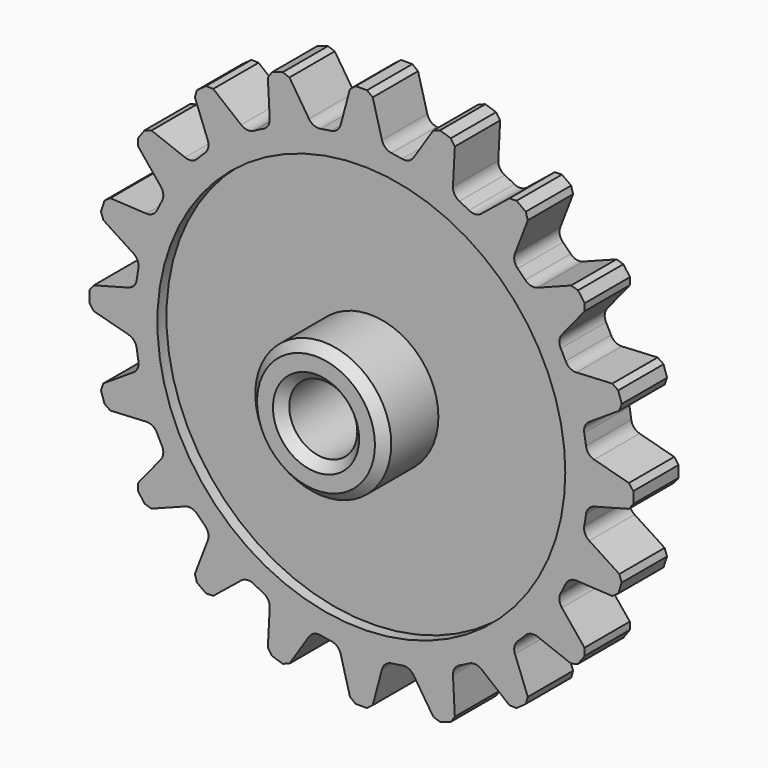
from build123d import *

# Parameters (mm, degrees)
F0_R            = 100
F1_DEPTH        = 25
F3_DEPTH        = 25
F3_COPIES_COUNT = 20
F4_R            = 5
F5_SIZE         = 2
F6_R            = 90
F7_DEPTH        = 5
F8_R            = 30
F9_DEPTH        = 30
F10_R           = 15
F11_DEPTH       = 50.001
F12_SIZE        = 4


# Not quite as in the source:
# - a pattern or mirror of a feature is missing from the dataset's text; its kind, count and spacing are read off the source's solid


with BuildPart() as f1:
    # F0 (on Front) → F1 (new body)
    with BuildSketch(Plane.XZ):
        Circle(F0_R)
    extrude(amount=F1_DEPTH)

    # F2 (on face) → F3 (join, through all)
    with BuildSketch(Plane.XZ.offset(25)):
        with BuildLine():
            Line((-4.5, 120), (-9.9931095726, 99.4994359837))
            ThreePointArc((-9.9931095726, 99.4994359837), (0, 100), (9.9931095726, 99.4994359837))
            Line((9.9931095726, 99.4994359837), (4.5, 120))
            Line((4.5, 120), (-4.5, 120))
        make_face()
    f3 = extrude(amount=-F3_DEPTH)

    # F3_copies: F3 ×20 about axis
    f3_copies_axis = Axis((0, 0, 0), (0, 1, 0))
    for i in range(1, F3_COPIES_COUNT):
        add(f3.rotate(f3_copies_axis, i * 360 / F3_COPIES_COUNT))

    # F4
    f4_edges = [f1.edges().sort_by_distance(p)[0] for p in [
        (9.99311, -12.5, 99.499436),
        (-9.99311, -12.5, 99.499436),
        (-21.243005, -12.5, 97.717628),
        (-50.399706, -12.5, 86.370537),
        (-40.251029, -12.5, 91.541546),
        (-66.568897, -12.5, 74.622932),
        (-74.622932, -12.5, 66.568897),
        (-86.370537, -12.5, 50.399706),
        (-91.541546, -12.5, 40.251029),
        (-97.717628, -12.5, 21.243005),
        (-99.499436, -12.5, 9.99311),
        (-99.499436, -12.5, -9.99311),
        (-97.717628, -12.5, -21.243005),
        (-91.541546, -12.5, -40.251029),
        (-86.370537, -12.5, -50.399706),
        (-74.622932, -12.5, -66.568897),
        (-66.568897, -12.5, -74.622932),
        (-50.399706, -12.5, -86.370537),
        (-40.251029, -12.5, -91.541546),
        (-21.243005, -12.5, -97.717628),
        (-9.99311, -12.5, -99.499436),
        (9.99311, -12.5, -99.499436),
        (21.243005, -12.5, -97.717628),
        (40.251029, -12.5, -91.541546),
        (50.399706, -12.5, -86.370537),
        (66.568897, -12.5, -74.622932),
        (74.622932, -12.5, -66.568897),
        (86.370537, -12.5, -50.399706),
        (91.541546, -12.5, -40.251029),
        (97.717628, -12.5, -21.243005),
        (99.499436, -12.5, -9.99311),
        (99.499436, -12.5, 9.99311),
        (97.717628, -12.5, 21.243005),
        (91.541546, -12.5, 40.251029),
        (86.370537, -12.5, 50.399706),
        (74.622932, -12.5, 66.568897),
        (66.568897, -12.5, 74.622932),
        (50.399706, -12.5, 86.370537),
        (40.251029, -12.5, 91.541546),
        (21.243005, -12.5, 97.717628),
    ]]
    fillet(f4_edges, radius=F4_R)

    # F5
    f5_edges = [f1.edges().sort_by_distance(p)[0] for p in [
        (4.5, -12.5, 120),
        (-4.5, -12.5, 120),
        (32.802285, -12.5, 115.517358),
        (41.361794, -12.5, 112.736205),
        (-32.802285, -12.5, 115.517358),
        (-41.361794, -12.5, 112.736205),
        (66.893654, -12.5, 99.727073),
        (74.174807, -12.5, 94.437006),
        (-66.893654, -12.5, 99.727073),
        (-74.174807, -12.5, 94.437006),
        (94.437006, -12.5, 74.174807),
        (99.727073, -12.5, 66.893654),
        (-94.437006, -12.5, 74.174807),
        (-99.727073, -12.5, 66.893654),
        (112.736205, -12.5, 41.361794),
        (115.517358, -12.5, 32.802285),
        (-112.736205, -12.5, 41.361794),
        (-115.517358, -12.5, 32.802285),
        (120, -12.5, 4.5),
        (120, -12.5, -4.5),
        (-120, -12.5, 4.5),
        (-120, -12.5, -4.5),
        (115.517358, -12.5, -32.802285),
        (112.736205, -12.5, -41.361794),
        (-115.517358, -12.5, -32.802285),
        (-112.736205, -12.5, -41.361794),
        (99.727073, -12.5, -66.893654),
        (94.437006, -12.5, -74.174807),
        (-99.727073, -12.5, -66.893654),
        (-94.437006, -12.5, -74.174807),
        (74.174807, -12.5, -94.437006),
        (66.893654, -12.5, -99.727073),
        (-74.174807, -12.5, -94.437006),
        (-66.893654, -12.5, -99.727073),
        (41.361794, -12.5, -112.736205),
        (32.802285, -12.5, -115.517358),
        (-41.361794, -12.5, -112.736205),
        (-32.802285, -12.5, -115.517358),
        (4.5, -12.5, -120),
        (-4.5, -12.5, -120),
    ]]
    chamfer(f5_edges, length=F5_SIZE)

    # F6 (on face) → F7 (cut)
    with BuildSketch(Plane.XZ.offset(25)):
        Circle(F6_R)
    extrude(amount=-F7_DEPTH, mode=Mode.SUBTRACT)

    # F8 (on face) → F9 (join)
    with BuildSketch(Plane.XZ.offset(20)):
        Circle(F8_R)
    extrude(amount=F9_DEPTH)

    # F10 (on face) → F11 (cut, through all)
    with BuildSketch(Plane.XZ.offset(50)):
        Circle(F10_R)
    extrude(amount=-F11_DEPTH, mode=Mode.SUBTRACT)

    # F12
    f12_edges = [f1.edges().sort_by_distance(p)[0] for p in [
        (-30, -50, 0),
        (-15, -50, 0),
    ]]
    chamfer(f12_edges, length=F12_SIZE)


solid = f1.part
